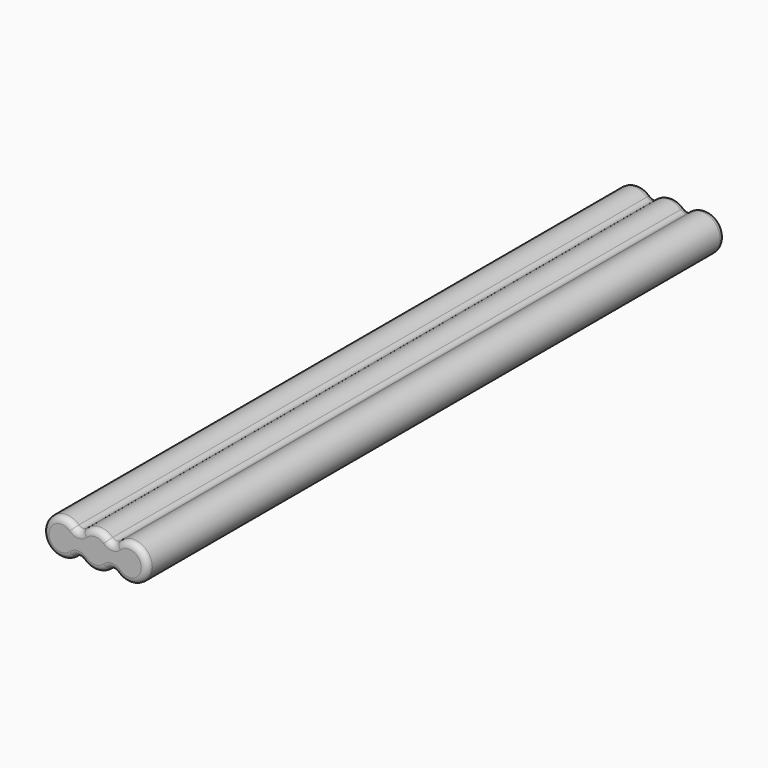
from build123d import *

# Parameters (mm, degrees)
F1_DEPTH = 74.6125
F2_R     = 1.27


with BuildPart() as f1:
    # F0 (on Front) → F1 (new body, symmetric)
    with BuildSketch(Plane.XZ):
        with BuildLine():
            ThreePointArc((-3.4925, -1.5226765087), (0, -3.81), (3.4925, -1.5226765087))
            ThreePointArc((3.4925, -1.5226765087), (10.795, 0), (3.4925, 1.5226765087))
            ThreePointArc((3.4925, 1.5226765087), (0, 3.81), (-3.4925, 1.5226765087))
            ThreePointArc((-3.4925, 1.5226765087), (-10.795, 0), (-3.4925, -1.5226765087))
        make_face()
    extrude(amount=F1_DEPTH, both=True)

    # F2
    f2_edges = [f1.edges().sort_by_distance(p)[0] for p in [
        (0, 74.6125, 3.81),
        (-3.4925, 0, 1.522677),
        (0, -74.6125, 3.81),
        (3.4925, 0, 1.522677),
        (10.795, 74.6125, 0),
        (10.795, -74.6125, 0),
        (3.4925, 0, -1.522677),
        (-10.795, 74.6125, 0),
        (-3.4925, 0, -1.522677),
        (-10.795, -74.6125, 0),
        (0, 74.6125, -3.81),
        (0, -74.6125, -3.81),
    ]]
    fillet(f2_edges, radius=F2_R)


solid = f1.part
